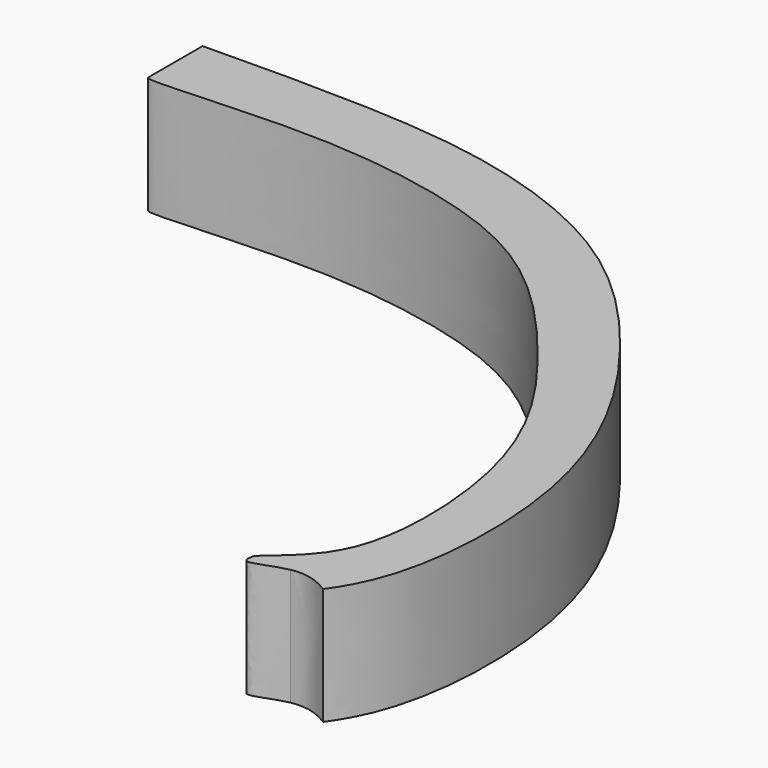
from build123d import *

# Parameters (mm, degrees)
F1_DEPTH = 25.4


with BuildPart() as f1:
    # F0 (on Top) → F1 (new body)
    with BuildSketch(Plane.XY):
        with BuildLine():
            add(Edge.make_bspline(
                [(0, 32.3620848358), (4.616245299, 36.3944720125), (15.4983274834, 44.6984201373), (13.6666682436, 88.8627259497), (-7.097495706, 119.4566531382), (-32.5079925777, 147.3610034027), (-62.5358454037, 156.9909503606), (-91.9306865929, 159.8354501402), (-120.8391481347, 157.3326324801), (-123.9743855546, 157.9896672991), (-123.8329410553, 158.3019942045)],
                knots=[0, 0, 0, 0, 0.1046496121, 0.2605304968, 0.4133735293, 0.5625949593, 0.6979575673, 0.8378718565, 0.9686560343, 1, 1, 1, 1], degree=3))
            add(Edge.make_bspline(
                [(7.9113617539, 32.1550443769), (4.7203534146, 31.5526155318), (-1.0409519817, 28.3342911106), (-0.2116711823, 31.5519841263), (0, 32.3620848358)],
                knots=[0.4072781194, 0.4072781194, 0.4072781194, 0.4072781194, 0.7956278657, 1, 1, 1, 1], degree=3))
            add(Edge.make_bspline(
                [(16.6635511817, 30.0982165935), (16.7030308183, 30.2622075198), (17.0150531463, 32.7150187131), (10.8724841867, 35.4521642858), (8.5677795334, 33.1385749466), (7.9113617539, 32.1550443769)],
                knots=[0.3546609767, 0.3546609767, 0.3546609767, 0.3546609767, 0.3617589695, 0.4623198499, 0.5097820379, 0.5097820379, 0.5097820379, 0.5097820379], degree=3))
            add(Edge.make_bspline(
                [(-123.8329410553, 172.9773198607), (-113.6918879881, 173.1962776362), (-92.015737529, 173.3126790169), (-60.3657998712, 171.4315667112), (-25.7083616084, 159.2218478032), (1.6611720718, 132.14191491), (27.1899010949, 91.1007415152), (26.0918092721, 45.9492515021), (18.6801450725, 32.8924904799), (16.6635511817, 30.0982165935)],
                knots=[0, 0, 0, 0, 0.1342724804, 0.2692810288, 0.4114531234, 0.5583310233, 0.72502551, 0.8912530752, 0.9464123607, 0.9464123607, 0.9464123607, 0.9464123607], degree=3))
            Line((-123.8329410553, 172.9773198607), (-123.8329410553, 158.3019942045))
        make_face()
        with BuildLine():
            add(Edge.make_bspline(
                [(16.6635511817, 30.0982165935), (16.7030308183, 30.2622075198), (17.0150531463, 32.7150187131), (10.8724841867, 35.4521642858), (8.5677795334, 33.1385749466), (7.9113617539, 32.1550443769)],
                knots=[0.3546609767, 0.3546609767, 0.3546609767, 0.3546609767, 0.3617589695, 0.4623198499, 0.5097820379, 0.5097820379, 0.5097820379, 0.5097820379], degree=3))
            add(Edge.make_bspline(
                [(16.6635511817, 30.0982165935), (13.9623635483, 31.7620139941), (11.2579015364, 32.7868359241), (7.9113617539, 32.1550443769)],
                knots=[0, 0, 0, 0, 0.4072781194, 0.4072781194, 0.4072781194, 0.4072781194], degree=3))
        make_face()
    extrude(amount=F1_DEPTH)


solid = f1.part
